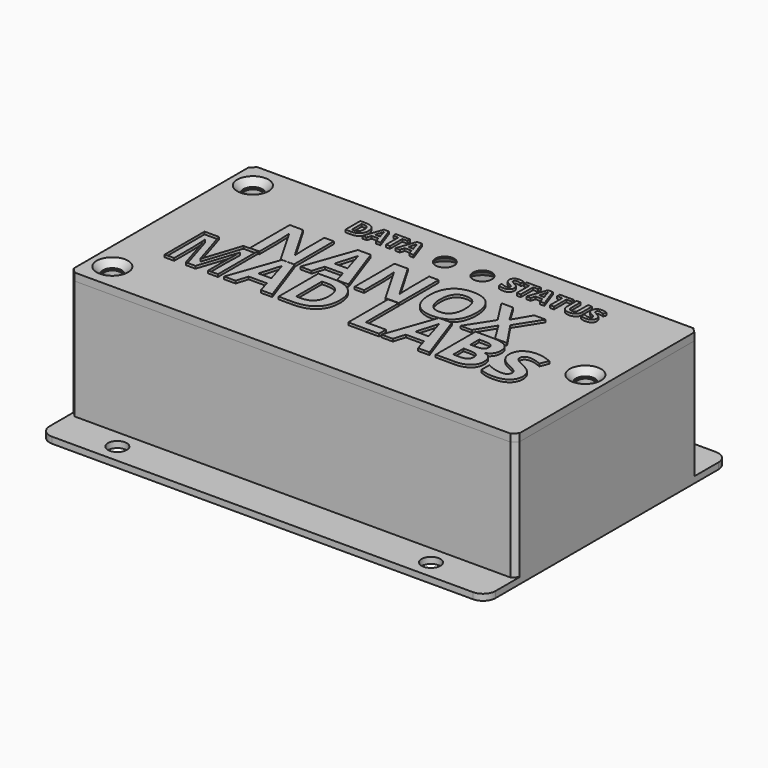
from build123d import *

# Parameters (mm, degrees)
F0_R            = 1.25
F1_DEPTH        = 19
F0_W            = 71.097931716
F0_H            = 6
F0_R_2          = 1.5
F2_DEPTH        = 1
F3_R            = 2
F4_SIZE         = 0.8
F5_R            = 2.5
F6_W            = 71.09793
F6_H            = 36.4
F6_R            = 1.5
F7_DEPTH        = 1.2
F8_SIZE         = 0.8
F9_SIZE         = 1
F10_TEXT_SIZE   = 11.1111111111
F10_TEXT_SIZE_2 = 4.1666666667
F11_DEPTH       = 0.4


# Not quite as in the source:
# - a feature names something its author has since deleted; it is built from what else it names
# - Text() gives the source's letters only with a copy of the font that has no kerning and outlines rounded to 1/6400 em; it was checked with that copy


with BuildPart() as f1:
    # F0 (on Top) → F1 (new body)
    with BuildSketch(Plane.XY):
        Polygon((0, 18.2), (0, 6), (71.097931716, 6), (71.097931716, 42.4), (0, 42.4), (0, 30.2), (1.2, 30.2), (1.2, 35.2), (5.7, 35.2), (5.7, 41.2), (69.897931716, 41.2), (69.897931716, 26.95), (65.397931716, 26.95), (65.397931716, 21.45), (69.897931716, 21.45), (69.897931716, 7.2), (5.7, 7.2), (5.7, 13.2), (1.2, 13.2), (1.2, 18.2), align=None)
        with Locations((3.45, 10.2)):
            Circle(F0_R, mode=Mode.SUBTRACT)
        with Locations((3.45, 38.2)):
            Circle(F0_R, mode=Mode.SUBTRACT)
        with Locations((67.647931716, 24.2)):
            Circle(F0_R, mode=Mode.SUBTRACT)
    extrude(amount=F1_DEPTH)

    # F0 (on Top) → F2 (join)
    with BuildSketch(Plane.XY):
        Polygon((0, 18.2), (0, 6), (71.097931716, 6), (71.097931716, 42.4), (0, 42.4), (0, 30.2), (1.2, 30.2), (1.2, 35.2), (5.7, 35.2), (5.7, 41.2), (69.897931716, 41.2), (69.897931716, 26.95), (65.397931716, 26.95), (65.397931716, 21.45), (69.897931716, 21.45), (69.897931716, 7.2), (5.7, 7.2), (5.7, 13.2), (1.2, 13.2), (1.2, 18.2), align=None)
        with Locations((3.45, 10.2)):
            Circle(F0_R, mode=Mode.SUBTRACT)
        with Locations((3.45, 38.2)):
            Circle(F0_R, mode=Mode.SUBTRACT)
        with Locations((67.647931716, 24.2)):
            Circle(F0_R, mode=Mode.SUBTRACT)
        with Locations((35.548965858, 3)):
            Rectangle(F0_W, F0_H)
        with Locations((10, 3)):
            Circle(F0_R_2, mode=Mode.SUBTRACT)
        with Locations((60, 3)):
            Circle(F0_R_2, mode=Mode.SUBTRACT)
        Polygon((0, 30.2), (0, 18.2), (1.2, 18.2), (1.2, 13.2), (5.7, 13.2), (5.7, 7.2), (69.897931716, 7.2), (69.897931716, 21.45), (65.397931716, 21.45), (65.397931716, 26.95), (69.897931716, 26.95), (69.897931716, 41.2), (5.7, 41.2), (5.7, 35.2), (1.2, 35.2), (1.2, 30.2), align=None)
        with Locations((35.548965858, 45.4)):
            Rectangle(F0_W, F0_H)
        with Locations((10, 45.4)):
            Circle(F0_R_2, mode=Mode.SUBTRACT)
        with Locations((60, 45.4)):
            Circle(F0_R_2, mode=Mode.SUBTRACT)
        with Locations((3.45, 10.2)):
            Circle(F0_R)
        with Locations((67.647931716, 24.2)):
            Circle(F0_R)
        with Locations((3.45, 38.2)):
            Circle(F0_R)
    extrude(amount=-F2_DEPTH)

    # F3
    f3_edges = [f1.edges().sort_by_distance(p)[0] for p in [
        (0, 0, -0.5),
        (71.097932, 0, -0.5),
        (71.097932, 48.4, -0.5),
        (0, 48.4, -0.5),
    ]]
    fillet(f3_edges, radius=F3_R)

    # F4
    f4_edges = [f1.edges().sort_by_distance(p)[0] for p in [
        (0, 42.4, 9.5),
        (0, 6, 9.5),
        (71.097932, 6, 9.5),
        (71.097932, 42.4, 9.5),
    ]]
    chamfer(f4_edges, length=F4_SIZE)

    # F5
    f5_edges = [f1.edges().sort_by_distance(p)[0] for p in [
        (5.7, 35.2, 9.5),
        (65.397932, 21.45, 9.5),
        (65.397932, 26.95, 9.5),
        (5.7, 13.2, 9.5),
    ]]
    fillet(f5_edges, radius=F5_R)


with BuildPart() as f7:
    # F6 (on face) → F7 (new body)
    with BuildSketch(Plane.XY.offset(19)):
        with Locations((35.548965, 24.2)):
            Rectangle(F6_W, F6_H)
        with Locations((3.45, 10.2)):
            Circle(F6_R, mode=Mode.SUBTRACT)
        with Locations((67.648, 24.2)):
            Circle(F6_R, mode=Mode.SUBTRACT)
        with Locations((3.45, 38.2)):
            Circle(F6_R, mode=Mode.SUBTRACT)
        with Locations((35, 37)):
            Circle(F6_R, mode=Mode.SUBTRACT)
        with Locations((41, 37)):
            Circle(F6_R, mode=Mode.SUBTRACT)
    extrude(amount=F7_DEPTH)

    # F8
    f8_edges = [f7.edges().sort_by_distance(p)[0] for p in [
        (0, 6, 19.6),
        (71.09793, 6, 19.6),
        (71.09793, 42.4, 19.6),
        (0, 42.4, 19.6),
    ]]
    chamfer(f8_edges, length=F8_SIZE)

    # F9
    f9_edges = [f7.edges().sort_by_distance(p)[0] for p in [
        (1.95, 10.2, 20.2),
        (1.95, 38.2, 20.2),
        (66.148, 24.2, 20.2),
        (39.5, 37, 19),
        (33.5, 37, 19),
    ]]
    chamfer(f9_edges, length=F9_SIZE)

    # F10 (on face) → F11 (join)
    with BuildSketch(Plane.XY.offset(20.2)):
        with Locations((13.175, 24.2)):
            Text('NANOX', F10_TEXT_SIZE, font='Open Sans', font_style=FontStyle.BOLD, text_align=(TextAlign.LEFT, TextAlign.BOTTOM))
        with Locations((6, 16.2)):
            Text('MAD LABS', F10_TEXT_SIZE, font='Open Sans', font_style=FontStyle.BOLD, text_align=(TextAlign.LEFT, TextAlign.BOTTOM))
        with Locations((19.982421875, 35.5)):
            Text('DATA', F10_TEXT_SIZE_2, font='Open Sans', font_style=FontStyle.BOLD, text_align=(TextAlign.LEFT, TextAlign.BOTTOM))
        with Locations((44.5, 35.5)):
            Text('STATUS', F10_TEXT_SIZE_2, font='Open Sans', font_style=FontStyle.BOLD, text_align=(TextAlign.LEFT, TextAlign.BOTTOM))
    extrude(amount=F11_DEPTH)


solid = Compound([f1.part, f7.part])
